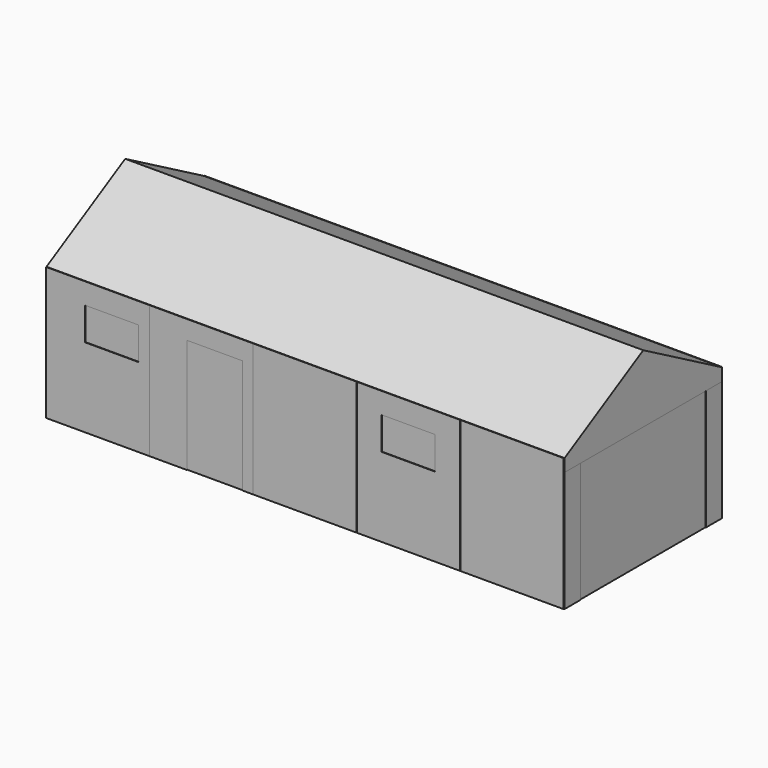
from build123d import *

# Parameters (mm, degrees)
F0_W        = 8000
F0_H        = 3040
F1_DEPTH    = 2055
F2_W        = 1596
F2_H        = 2055
F3_DEPTH    = 8
F4_W        = 310
F4_H        = 1860
F5_DEPTH    = 8
F6_W        = 1596
F6_H        = 2055
F7_DEPTH    = 8
F8_W        = 825
F8_H        = 505
F8_W_2      = 860
F8_H_2      = 1800
F9_DEPTH    = 8
F10_DEPTH   = 850
F11_SIZE2   = 849.99999
F11_SIZE    = 1519.99999
F12_W       = 3040
F12_H       = 1045
F13_DEPTH   = 8
F14_SIZE2   = 1520
F14_SIZE    = 850
F14_2_SIZE2 = 1519.99999
F14_2_SIZE  = 849.99999


# Not quite as in the source:
# - a fillet or chamfer is up to 0.001 mm smaller than in the source, because OpenCascade refuses the exact size


with BuildPart() as f1:
    # F0 (on Top) → F1 (new body)
    with BuildSketch(Plane.XY):
        Rectangle(F0_W, F0_H)
    extrude(amount=F1_DEPTH)


with BuildPart() as f3:
    # F2 (on face) → F3 (new body)
    with BuildSketch(Plane.XZ.offset(1520)):
        with Locations((3202, 1027.5)):
            Rectangle(F2_W, F2_H)
    extrude(amount=F3_DEPTH)


with BuildPart() as f3b:
    # F2 (on face) → F3, piece 2 (new body)
    with BuildSketch(Plane.XZ.offset(1520)):
        with Locations((1601, 1027.5)):
            Rectangle(F2_W, F2_H)
    extrude(amount=F3_DEPTH)


with BuildPart() as f3c:
    # F2 (on face) → F3, piece 3 (new body)
    with BuildSketch(Plane.XZ.offset(1520)):
        with Locations((0, 1027.5)):
            Rectangle(F2_W, F2_H)
    extrude(amount=F3_DEPTH)


with BuildPart() as f3d:
    # F2 (on face) → F3, piece 4 (new body)
    with BuildSketch(Plane.XZ.offset(1520)):
        with Locations((-1601, 1027.5)):
            Rectangle(F2_W, F2_H)
    extrude(amount=F3_DEPTH)


with BuildPart() as f3e:
    # F2 (on face) → F3, piece 5 (new body)
    with BuildSketch(Plane.XZ.offset(1520)):
        with Locations((-3202, 1027.5)):
            Rectangle(F2_W, F2_H)
    extrude(amount=F3_DEPTH)


with BuildPart() as f5:
    # F4 (on face) → F5 (new body)
    with BuildSketch(Plane.YZ.offset(4000)):
        with Locations((-1365, 930)):
            Rectangle(F4_W, F4_H)
    extrude(amount=F5_DEPTH)


with BuildPart() as f5b:
    # F4 (on face) → F5, piece 2 (new body)
    with BuildSketch(Plane.YZ.offset(4000)):
        with Locations((1365, 930)):
            Rectangle(F4_W, F4_H)
    extrude(amount=F5_DEPTH)


with BuildPart() as f7:
    # F6 (on face) → F7 (new body)
    with BuildSketch(Plane(origin=(0, 1520, 0), x_dir=(-1, 0, 0), z_dir=(0, 1, 0))):
        with Locations((-3202, 1027.5)):
            Rectangle(F6_W, F6_H)
    extrude(amount=F7_DEPTH)


with BuildPart() as f7b:
    # F6 (on face) → F7, piece 2 (new body)
    with BuildSketch(Plane(origin=(0, 1520, 0), x_dir=(-1, 0, 0), z_dir=(0, 1, 0))):
        with Locations((-1601, 1027.5)):
            Rectangle(F6_W, F6_H)
    extrude(amount=F7_DEPTH)


with BuildPart() as f7c:
    # F6 (on face) → F7, piece 3 (new body)
    with BuildSketch(Plane(origin=(0, 1520, 0), x_dir=(-1, 0, 0), z_dir=(0, 1, 0))):
        with Locations((0, 1027.5)):
            Rectangle(F6_W, F6_H)
    extrude(amount=F7_DEPTH)


with BuildPart() as f7d:
    # F6 (on face) → F7, piece 4 (new body)
    with BuildSketch(Plane(origin=(0, 1520, 0), x_dir=(-1, 0, 0), z_dir=(0, 1, 0))):
        with Locations((1601, 1027.5)):
            Rectangle(F6_W, F6_H)
    extrude(amount=F7_DEPTH)


with BuildPart() as f7e:
    # F6 (on face) → F7, piece 5 (new body)
    with BuildSketch(Plane(origin=(0, 1520, 0), x_dir=(-1, 0, 0), z_dir=(0, 1, 0))):
        with Locations((3202, 1027.5)):
            Rectangle(F6_W, F6_H)
    extrude(amount=F7_DEPTH)


with BuildPart() as f9_tool:
    # F8 (on face) → F9 (new body)
    with BuildSketch(Plane.XZ.offset(1520)):
        with Locations((1595.5, 1477.5)):
            Rectangle(F8_W, F8_H)
        with Locations((-2987.5, 1477.5)):
            Rectangle(F8_W, F8_H)
        with Locations((-1395, 865)):
            Rectangle(F8_W_2, F8_H_2)
    extrude(amount=F9_DEPTH)


with BuildPart() as f3b_1:
    add(f3b.part)

    # F9: cut by f9_tool
    add(f9_tool.part, mode=Mode.SUBTRACT)


with BuildPart() as f3d_1:
    add(f3d.part)

    # F9: cut by f9_tool
    add(f9_tool.part, mode=Mode.SUBTRACT)


with BuildPart() as f3e_1:
    add(f3e.part)

    # F9: cut by f9_tool
    add(f9_tool.part, mode=Mode.SUBTRACT)


with BuildPart() as f10:
    # F10 (new): a face of the model
    f10_faces = [f1.part.faces().sort_by_distance(p)[0] for p in [
        (0, 0, 2055),
    ]]
    extrude(f10_faces, amount=F10_DEPTH)

    # F11 (size 1520 and 850 in the source; OpenCascade refuses exactly that, so slightly less here)
    f11_edges = [f10.edges().sort_by_distance(p)[0] for p in [
        (0, -1520, 2905),
        (0, 1520, 2905),
    ]]
    f11_side = f10.faces().sort_by_distance((0, 0, 2905))[0]
    chamfer(f11_edges, length=F11_SIZE, length2=F11_SIZE2, reference=f11_side)


with BuildPart() as f13:
    # F12 (on face) → F13 (new body)
    with BuildSketch(Plane.YZ.offset(4000)):
        with Locations((0, 2382.5)):
            Rectangle(F12_W, F12_H)
    extrude(amount=F13_DEPTH)

    # F14
    f14_edges = [f13.edges().sort_by_distance(p)[0] for p in [
        (4004, -1520, 2905),
    ]]
    f14_side = f13.faces().sort_by_distance((4004, -1520, 2382.5))[0]
    chamfer(f14_edges, length=F14_SIZE, length2=F14_SIZE2, reference=f14_side)

    # F14#2 (size 850 and 1520 in the source; OpenCascade refuses exactly that, so slightly less here)
    f14_2_edges = [f13.edges().sort_by_distance(p)[0] for p in [
        (4004, 1520, 2905),
    ]]
    f14_2_side = f13.faces().sort_by_distance((4004, 1520, 2382.5))[0]
    chamfer(f14_2_edges, length=F14_2_SIZE, length2=F14_2_SIZE2, reference=f14_2_side)


solid = Compound([f1.part, f3.part, f3c.part, f5.part, f5b.part, f7.part, f7b.part, f7c.part, f7d.part, f7e.part, f3b_1.part, f3d_1.part, f3e_1.part, f10.part, f13.part])
